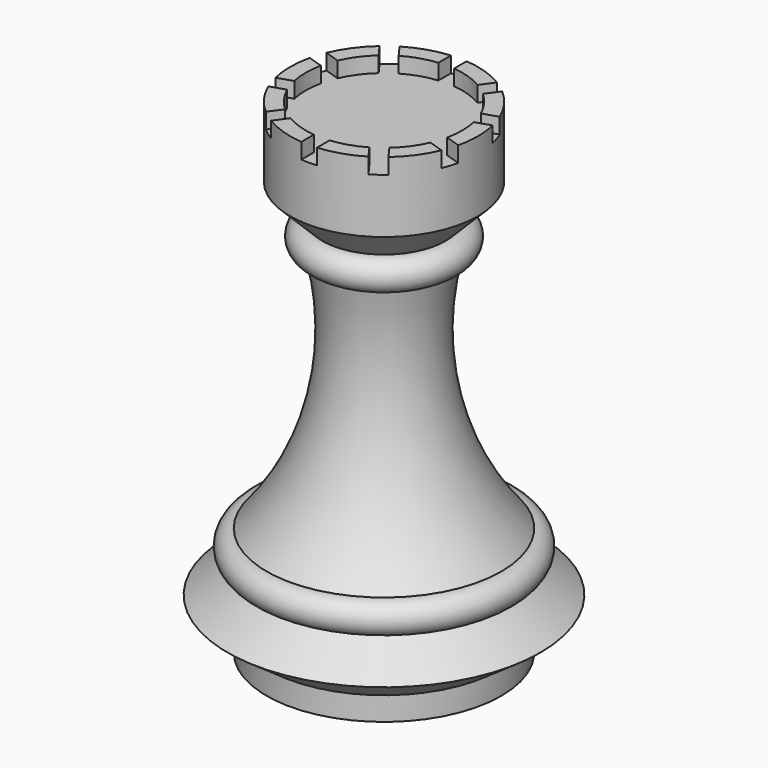
from build123d import *

# Parameters (mm, degrees)
F2_W            = 2.54
F2_H            = 2.54
F3_DEPTH        = 25.401
F3_DEPTH_BACK   = 25.401
F3_COPIES_COUNT = 5
F3_COPIES_ANGLE = 144


# Not quite as in the source:
# - a pattern or mirror of a feature is missing from the dataset's text; its kind, count and spacing are read off the source's solid


with BuildPart() as f1:
    # F0 (on Front) → F1 (revolve)
    with BuildSketch(Plane.XZ):
        with BuildLine():
            Line((0, 76.2), (0, 0))
            Line((0, 0), (19.05, 0))
            Line((19.05, 0), (19.05, 3.81))
            Line((19.05, 3.81), (25.4, 8.255))
            Line((25.4, 8.255), (19.05, 12.7))
            ThreePointArc((19.05, 12.7), (21.59, 15.24), (19.05, 17.78))
            ThreePointArc((19.05, 17.78), (9.8357933439, 36.306429206), (10.0070276085, 56.9970276085))
            ThreePointArc((10.0070276085, 56.9970276085), (12.5470276085, 59.5370276085), (10.0070276085, 62.0770276085))
            Line((10.0070276085, 62.0770276085), (15.24, 67.31))
            Line((15.24, 67.31), (15.24, 78.74))
            Line((15.24, 78.74), (12.7, 78.74))
            Line((12.7, 78.74), (12.7, 76.2))
            Line((12.7, 76.2), (0, 76.2))
        make_face()
    revolve(axis=Axis((0, 0, 38.1), (0, 0, 1)))

    # F2 (on Front) → F3 (cut, two sides)
    with BuildSketch(Plane.XZ) as f3_sk:
        with Locations((0, 77.47)):
            Rectangle(F2_W, F2_H)
    f3 = extrude(amount=-F3_DEPTH, mode=Mode.SUBTRACT) + extrude(f3_sk.sketch, amount=F3_DEPTH_BACK, mode=Mode.SUBTRACT)

    # F3_copies: F3 ×5 about axis
    f3_copies_axis = Axis((0, 0, 0), (0, 0, 1))
    for i in range(1, F3_COPIES_COUNT):
        add(f3.rotate(f3_copies_axis, i * F3_COPIES_ANGLE / (F3_COPIES_COUNT - 1)), mode=Mode.SUBTRACT)


solid = f1.part
